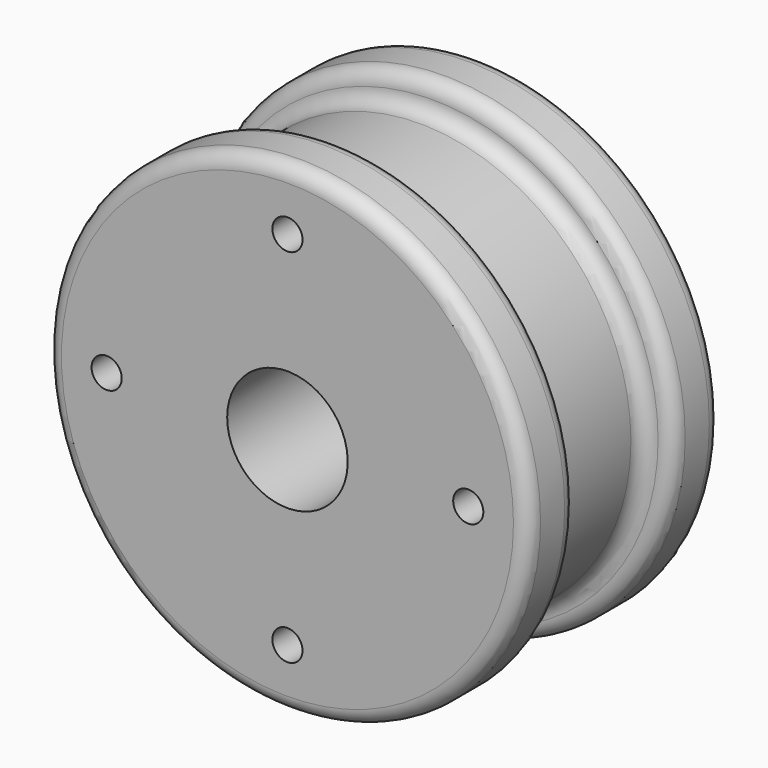
from build123d import *

# Parameters (mm, degrees)
F0_R     = 25.4
F1_DEPTH = 6.35
F2_R     = 22.225
F3_DEPTH = 12.7
F4_R     = 25.4
F5_DEPTH = 6.35
F6_R     = 1.58749
F8_D     = 3.175
F8_DEPTH = 3.175
F8_TIP   = 0.9538662327
F9_D     = 12.7


# Not quite as in the source:
# - a fillet or chamfer is up to 0.001 mm smaller than in the source, because OpenCascade refuses the exact size


with BuildPart() as f1:
    # F0 (on Front) → F1 (new body)
    with BuildSketch(Plane.XZ):
        Circle(F0_R)
    extrude(amount=F1_DEPTH)

    # F2 (on face) → F3 (join)
    with BuildSketch(Plane.XZ.offset(6.35)):
        Circle(F2_R)
    extrude(amount=F3_DEPTH)

    # F4 (on face) → F5 (join)
    with BuildSketch(Plane.XZ.offset(19.05)):
        Circle(F4_R)
    extrude(amount=F5_DEPTH)

    # F6 (radius 1.5875 in the source; OpenCascade refuses exactly that, so slightly less here)
    f6_edges = [f1.edges().sort_by_distance(p)[0] for p in [
        (-25.4, 0, 0),
        (-25.4, -6.35, 0),
        (-25.4, -25.4, 0),
        (-25.4, -19.05, 0),
        (-22.225, -19.05, 0),
        (-22.225, -6.35, 0),
    ]]
    fillet(f6_edges, radius=F6_R)

    # F8
    with Locations(Plane.XZ.offset(25.4)):
        with Locations((0, 19.05), (19.05, 0), (0, -19.05), (-19.05, 0)):
            Hole(F8_D / 2, depth=F8_DEPTH)
            with Locations((0, 0, -(F8_DEPTH + F8_TIP / 2))):  # 118° drill point
                Cone(0, F8_D / 2, F8_TIP, mode=Mode.SUBTRACT)

    # F9 (through all)
    with Locations(Plane.XZ.offset(25.4)):
        with Locations((0, 0)):
            Hole(F9_D / 2)


solid = f1.part
